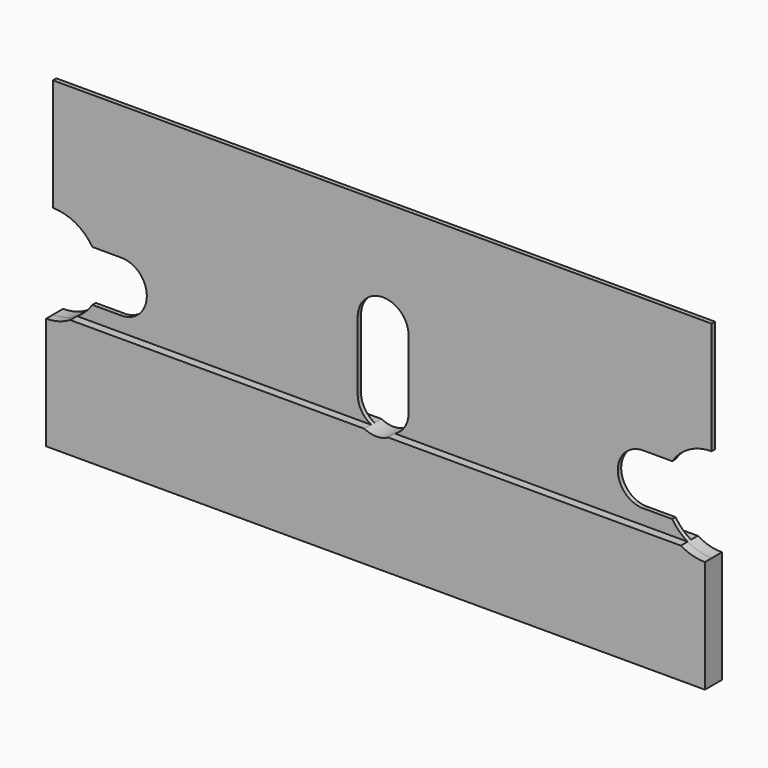
from build123d import *

# Parameters (mm, degrees)
F1_DEPTH = 0.254
F3_DEPTH = 0.508
F4_DEPTH = 1.27


# Not quite as in the source:
# - a feature of the source that left no trace in its solid (it failed there, or was rolled back) is left out


with BuildPart() as f1:
    # F0 (on Front) → F1 (new body)
    with BuildSketch(Plane.XZ):
        with BuildLine():
            Line((-19.685, -9.525), (19.685, -9.525))
            Line((19.685, -9.525), (19.685, -2.8099691571))
            ThreePointArc((19.685, -2.8099691571), (18.3397695065, -2.4670390316), (17.3228842981, -1.5219514036))
            Line((17.3228842981, -1.5219514036), (15.6737824523, -1.5219514036))
            ThreePointArc((15.6737824523, -1.5219514036), (14.0708501874, -0.0136277742), (15.6465519968, 1.5231206842))
            Line((15.6465519968, 1.5231206842), (17.3222628429, 1.5209864531))
            ThreePointArc((17.3222628429, 1.5209864531), (18.3392656944, 2.4667642455), (19.685, 2.8099691571))
            Line((19.685, 2.8099691571), (19.685, 9.525))
            Line((19.685, 9.525), (-19.685, 9.525))
            Line((-19.685, 9.525), (-19.685, 2.8099691571))
            ThreePointArc((-19.685, 2.8099691571), (-18.3392656944, 2.4667642455), (-17.3222628429, 1.5209864531))
            Line((-17.3222628429, 1.5209864531), (-15.6465519968, 1.5231206842))
            ThreePointArc((-15.6465519968, 1.5231206842), (-14.0708501874, -0.0136277742), (-15.6737824523, -1.5219514036))
            Line((-15.6737824523, -1.5219514036), (-17.3228842981, -1.5219514036))
            ThreePointArc((-17.3228842981, -1.5219514036), (-18.3397695065, -2.4670390316), (-19.685, -2.8099691571))
            Line((-19.685, -2.8099691571), (-19.685, -9.525))
        make_face()
        with BuildLine():
            Line((1.5744257675, 2.9995050863), (1.5744257675, -1.0644949137))
            ThreePointArc((1.5744257675, -1.0644949137), (1.1189219615, -2.1511834079), (0.0246988863, -2.5882777484))
            ThreePointArc((0.0246988863, -2.5882777484), (-1.0362627267, -2.1329911076), (-1.4735742325, -1.0644949137))
            Line((-1.4735742325, -1.0644949137), (-1.4735742325, 2.9995050863))
            ThreePointArc((-1.4735742325, 2.9995050863), (-1.0670804368, 4.035727014), (-0.0644457766, 4.5191696968))
            ThreePointArc((-0.0644457766, 4.5191696968), (-0.0070508957, 4.5224208533), (0.0504257675, 4.5235050863))
            ThreePointArc((0.0504257675, 4.5235050863), (1.1280565021, 4.0771358209), (1.5744257675, 2.9995050863))
        make_face(mode=Mode.SUBTRACT)
    extrude(amount=F1_DEPTH)

    # F2 (on face) → F3 (join)
    with BuildSketch(Plane.XZ.offset(0.254)):
        with BuildLine():
            Line((-19.685, -2.8099691571), (-19.685, -9.525))
            Line((-19.685, -9.525), (19.685, -9.525))
            Line((19.685, -9.525), (19.685, -2.8099691571))
            ThreePointArc((19.685, -2.8099691571), (18.9381830586, -2.7089095814), (18.2450841469, -2.413))
            Line((18.2450841469, -2.413), (0.7604328323, -2.413))
            ThreePointArc((0.7604328323, -2.413), (0.0504257675, -2.5884949137), (-0.6595812973, -2.413))
            Line((-0.6595812973, -2.413), (-18.2450841469, -2.413))
            ThreePointArc((-18.2450841469, -2.413), (-18.9381830586, -2.7089095814), (-19.685, -2.8099691571))
        make_face()
    extrude(amount=F3_DEPTH)

    # F4 (add): a face of the model
    f4_faces = [f1.faces().sort_by_distance(p)[0] for p in [
        (-3.03846e-05, -0.762, -5.9805151068),
    ]]
    extrude(f4_faces, amount=-F4_DEPTH)


with BuildPart() as f6_1:
    # F6: copy of F1
    add(f1.part)


solid = Compound([f1.part, f6_1.part])
